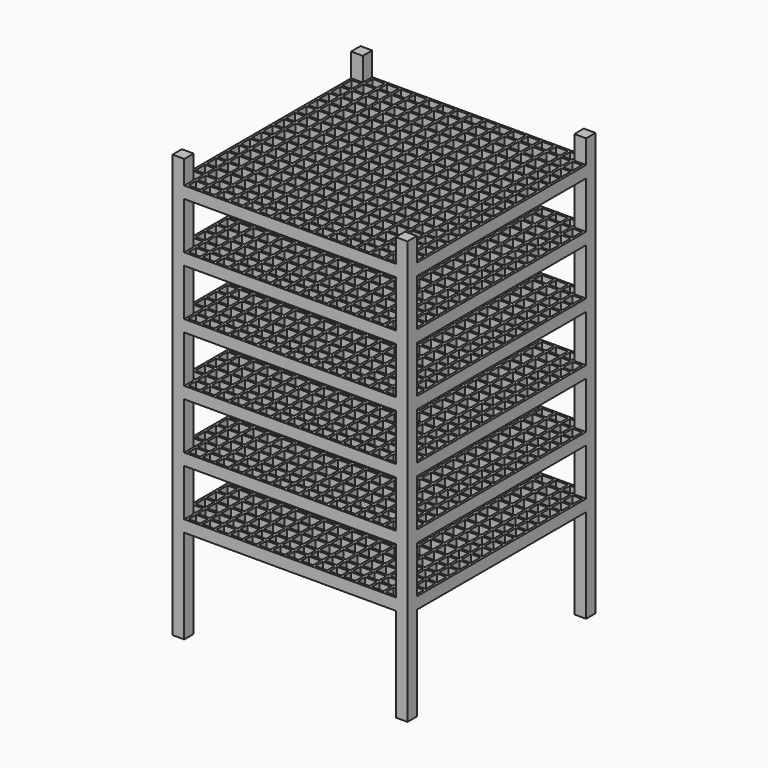
from build123d import *

# Parameters (mm, degrees)
F0_W     = 1000
F0_H     = 1000
F1_DEPTH = 1800
F2_W     = 900
F2_H     = 400
F2_H_2   = 200
F2_H_3   = 100
F4_DEPTH = 1000
F3_W     = 900
F3_H     = 400
F3_H_2   = 200
F3_H_3   = 100
F5_DEPTH = 1000
F6_W     = 40
F6_H     = 40
F6_H_2   = 50
F6_H_3   = 39.9711348116
F6_W_2   = 50
F7_DEPTH = 1800


with BuildPart() as f1:
    # F0 (on Top) → F1 (new body)
    with BuildSketch(Plane.XY):
        with Locations((-500, 500)):
            Rectangle(F0_W, F0_H)
    extrude(amount=F1_DEPTH)

    # F2 (on face) → F4 (cut)
    with BuildSketch(Plane.XZ):
        with Locations((-500, 200)):
            Rectangle(F2_W, F2_H)
        with Locations((-500, 550)):
            Rectangle(F2_W, F2_H_2)
        with Locations((-500, 800)):
            Rectangle(F2_W, F2_H_2)
        with Locations((-500, 1050)):
            Rectangle(F2_W, F2_H_2)
        with Locations((-500, 1300)):
            Rectangle(F2_W, F2_H_2)
        with Locations((-500, 1550)):
            Rectangle(F2_W, F2_H_2)
        with Locations((-500, 1750)):
            Rectangle(F2_W, F2_H_3)
    extrude(amount=-F4_DEPTH, mode=Mode.SUBTRACT)

    # F3 (on face) → F5 (cut)
    with BuildSketch(Plane.YZ):
        with Locations((500, 200)):
            Rectangle(F3_W, F3_H)
        with Locations((500, 550)):
            Rectangle(F3_W, F3_H_2)
        with Locations((500, 800)):
            Rectangle(F3_W, F3_H_2)
        with Locations((500, 1050)):
            Rectangle(F3_W, F3_H_2)
        with Locations((500, 1300)):
            Rectangle(F3_W, F3_H_2)
        with Locations((500, 1550)):
            Rectangle(F3_W, F3_H_2)
        with Locations((500, 1750)):
            Rectangle(F3_W, F3_H_3)
    extrude(amount=-F5_DEPTH, mode=Mode.SUBTRACT)

    # F6 (on face) → F7 (cut)
    with BuildSketch(Plane.XY.offset(1700)):
        with Locations((-30, 80)):
            Rectangle(F6_W, F6_H)
        with Locations((-30, 915)):
            Rectangle(F6_W, F6_H_2)
        with Locations((-30, 855)):
            Rectangle(F6_W, F6_H_2)
        with Locations((-30, 795)):
            Rectangle(F6_W, F6_H_2)
        with Locations((-30, 735)):
            Rectangle(F6_W, F6_H_2)
        with Locations((-30, 675)):
            Rectangle(F6_W, F6_H_2)
        with Locations((-30, 615)):
            Rectangle(F6_W, F6_H_2)
        with Locations((-30, 555)):
            Rectangle(F6_W, F6_H_2)
        with Locations((-30, 495)):
            Rectangle(F6_W, F6_H_2)
        with Locations((-30, 435)):
            Rectangle(F6_W, F6_H_2)
        with Locations((-30, 375)):
            Rectangle(F6_W, F6_H_2)
        with Locations((-30, 315)):
            Rectangle(F6_W, F6_H_2)
        with Locations((-30, 255)):
            Rectangle(F6_W, F6_H_2)
        with Locations((-30, 195)):
            Rectangle(F6_W, F6_H_2)
        with Locations((-30, 135)):
            Rectangle(F6_W, F6_H_2)
        with Locations((-80, 30.0144325942)):
            Rectangle(F6_W, F6_H_3)
        with Locations((-80, 80)):
            Rectangle(F6_W, F6_H)
        with Locations((-80, 135)):
            Rectangle(F6_W, F6_H_2)
        with Locations((-80, 195)):
            Rectangle(F6_W, F6_H_2)
        with Locations((-80, 255)):
            Rectangle(F6_W, F6_H_2)
        with Locations((-80, 315)):
            Rectangle(F6_W, F6_H_2)
        with Locations((-80, 375)):
            Rectangle(F6_W, F6_H_2)
        with Locations((-80, 435)):
            Rectangle(F6_W, F6_H_2)
        with Locations((-80, 495)):
            Rectangle(F6_W, F6_H_2)
        with Locations((-80, 555)):
            Rectangle(F6_W, F6_H_2)
        with Locations((-80, 615)):
            Rectangle(F6_W, F6_H_2)
        with Locations((-80, 675)):
            Rectangle(F6_W, F6_H_2)
        with Locations((-80, 735)):
            Rectangle(F6_W, F6_H_2)
        with Locations((-80, 795)):
            Rectangle(F6_W, F6_H_2)
        with Locations((-80, 855)):
            Rectangle(F6_W, F6_H_2)
        with Locations((-80, 915)):
            Rectangle(F6_W, F6_H_2)
        with Locations((-80, 970)):
            Rectangle(F6_W, F6_H)
        with Locations((-135, 970)):
            Rectangle(F6_W_2, F6_H)
        with Locations((-135, 915)):
            Rectangle(F6_W_2, F6_H_2)
        with Locations((-135, 855)):
            Rectangle(F6_W_2, F6_H_2)
        with Locations((-135, 795)):
            Rectangle(F6_W_2, F6_H_2)
        with Locations((-135, 735)):
            Rectangle(F6_W_2, F6_H_2)
        with Locations((-135, 675)):
            Rectangle(F6_W_2, F6_H_2)
        with Locations((-135, 615)):
            Rectangle(F6_W_2, F6_H_2)
        with Locations((-135, 555)):
            Rectangle(F6_W_2, F6_H_2)
        with Locations((-135, 495)):
            Rectangle(F6_W_2, F6_H_2)
        with Locations((-135, 435)):
            Rectangle(F6_W_2, F6_H_2)
        with Locations((-135, 375)):
            Rectangle(F6_W_2, F6_H_2)
        with Locations((-135, 315)):
            Rectangle(F6_W_2, F6_H_2)
        with Locations((-135, 255)):
            Rectangle(F6_W_2, F6_H_2)
        with Locations((-135, 195)):
            Rectangle(F6_W_2, F6_H_2)
        with Locations((-135, 135)):
            Rectangle(F6_W_2, F6_H_2)
        with Locations((-135, 80)):
            Rectangle(F6_W_2, F6_H)
        with Locations((-135, 30.0144325942)):
            Rectangle(F6_W_2, F6_H_3)
        with Locations((-195, 30.0144325942)):
            Rectangle(F6_W_2, F6_H_3)
        with Locations((-195, 80)):
            Rectangle(F6_W_2, F6_H)
        with Locations((-195, 135)):
            Rectangle(F6_W_2, F6_H_2)
        with Locations((-195, 195)):
            Rectangle(F6_W_2, F6_H_2)
        with Locations((-195, 255)):
            Rectangle(F6_W_2, F6_H_2)
        with Locations((-195, 315)):
            Rectangle(F6_W_2, F6_H_2)
        with Locations((-195, 375)):
            Rectangle(F6_W_2, F6_H_2)
        with Locations((-195, 435)):
            Rectangle(F6_W_2, F6_H_2)
        with Locations((-195, 495)):
            Rectangle(F6_W_2, F6_H_2)
        with Locations((-195, 555)):
            Rectangle(F6_W_2, F6_H_2)
        with Locations((-195, 615)):
            Rectangle(F6_W_2, F6_H_2)
        with Locations((-195, 675)):
            Rectangle(F6_W_2, F6_H_2)
        with Locations((-195, 735)):
            Rectangle(F6_W_2, F6_H_2)
        with Locations((-195, 795)):
            Rectangle(F6_W_2, F6_H_2)
        with Locations((-195, 855)):
            Rectangle(F6_W_2, F6_H_2)
        with Locations((-195, 915)):
            Rectangle(F6_W_2, F6_H_2)
        with Locations((-255, 970)):
            Rectangle(F6_W_2, F6_H)
        with Locations((-195, 970)):
            Rectangle(F6_W_2, F6_H)
        with Locations((-255, 915)):
            Rectangle(F6_W_2, F6_H_2)
        with Locations((-255, 855)):
            Rectangle(F6_W_2, F6_H_2)
        with Locations((-255, 795)):
            Rectangle(F6_W_2, F6_H_2)
        with Locations((-255, 735)):
            Rectangle(F6_W_2, F6_H_2)
        with Locations((-255, 675)):
            Rectangle(F6_W_2, F6_H_2)
        with Locations((-255, 615)):
            Rectangle(F6_W_2, F6_H_2)
        with Locations((-255, 555)):
            Rectangle(F6_W_2, F6_H_2)
        with Locations((-255, 495)):
            Rectangle(F6_W_2, F6_H_2)
        with Locations((-255, 435)):
            Rectangle(F6_W_2, F6_H_2)
        with Locations((-255, 375)):
            Rectangle(F6_W_2, F6_H_2)
        with Locations((-255, 315)):
            Rectangle(F6_W_2, F6_H_2)
        with Locations((-255, 255)):
            Rectangle(F6_W_2, F6_H_2)
        with Locations((-255, 195)):
            Rectangle(F6_W_2, F6_H_2)
        with Locations((-255, 135)):
            Rectangle(F6_W_2, F6_H_2)
        with Locations((-255, 80)):
            Rectangle(F6_W_2, F6_H)
        with Locations((-255, 30.0144325942)):
            Rectangle(F6_W_2, F6_H_3)
        with Locations((-315, 30.0144325942)):
            Rectangle(F6_W_2, F6_H_3)
        with Locations((-315, 80)):
            Rectangle(F6_W_2, F6_H)
        with Locations((-315, 135)):
            Rectangle(F6_W_2, F6_H_2)
        with Locations((-315, 195)):
            Rectangle(F6_W_2, F6_H_2)
        with Locations((-315, 255)):
            Rectangle(F6_W_2, F6_H_2)
        with Locations((-315, 315)):
            Rectangle(F6_W_2, F6_H_2)
        with Locations((-315, 375)):
            Rectangle(F6_W_2, F6_H_2)
        with Locations((-315, 435)):
            Rectangle(F6_W_2, F6_H_2)
        with Locations((-315, 495)):
            Rectangle(F6_W_2, F6_H_2)
        with Locations((-315, 555)):
            Rectangle(F6_W_2, F6_H_2)
        with Locations((-315, 615)):
            Rectangle(F6_W_2, F6_H_2)
        with Locations((-315, 675)):
            Rectangle(F6_W_2, F6_H_2)
        with Locations((-315, 735)):
            Rectangle(F6_W_2, F6_H_2)
        with Locations((-315, 795)):
            Rectangle(F6_W_2, F6_H_2)
        with Locations((-315, 855)):
            Rectangle(F6_W_2, F6_H_2)
        with Locations((-315, 915)):
            Rectangle(F6_W_2, F6_H_2)
        with Locations((-315, 970)):
            Rectangle(F6_W_2, F6_H)
        with Locations((-375, 970)):
            Rectangle(F6_W_2, F6_H)
        with Locations((-375, 915)):
            Rectangle(F6_W_2, F6_H_2)
        with Locations((-375, 855)):
            Rectangle(F6_W_2, F6_H_2)
        with Locations((-375, 795)):
            Rectangle(F6_W_2, F6_H_2)
        with Locations((-375, 735)):
            Rectangle(F6_W_2, F6_H_2)
        with Locations((-375, 675)):
            Rectangle(F6_W_2, F6_H_2)
        with Locations((-375, 615)):
            Rectangle(F6_W_2, F6_H_2)
        with Locations((-375, 555)):
            Rectangle(F6_W_2, F6_H_2)
        with Locations((-375, 495)):
            Rectangle(F6_W_2, F6_H_2)
        with Locations((-375, 435)):
            Rectangle(F6_W_2, F6_H_2)
        with Locations((-375, 375)):
            Rectangle(F6_W_2, F6_H_2)
        with Locations((-375, 315)):
            Rectangle(F6_W_2, F6_H_2)
        with Locations((-375, 255)):
            Rectangle(F6_W_2, F6_H_2)
        with Locations((-375, 195)):
            Rectangle(F6_W_2, F6_H_2)
        with Locations((-375, 135)):
            Rectangle(F6_W_2, F6_H_2)
        with Locations((-375, 80)):
            Rectangle(F6_W_2, F6_H)
        with Locations((-375, 30.0144325942)):
            Rectangle(F6_W_2, F6_H_3)
        with Locations((-435, 30.0144325942)):
            Rectangle(F6_W_2, F6_H_3)
        with Locations((-435, 80)):
            Rectangle(F6_W_2, F6_H)
        with Locations((-435, 135)):
            Rectangle(F6_W_2, F6_H_2)
        with Locations((-435, 195)):
            Rectangle(F6_W_2, F6_H_2)
        with Locations((-435, 255)):
            Rectangle(F6_W_2, F6_H_2)
        with Locations((-435, 315)):
            Rectangle(F6_W_2, F6_H_2)
        with Locations((-435, 375)):
            Rectangle(F6_W_2, F6_H_2)
        with Locations((-435, 435)):
            Rectangle(F6_W_2, F6_H_2)
        with Locations((-435, 495)):
            Rectangle(F6_W_2, F6_H_2)
        with Locations((-435, 555)):
            Rectangle(F6_W_2, F6_H_2)
        with Locations((-435, 615)):
            Rectangle(F6_W_2, F6_H_2)
        with Locations((-435, 675)):
            Rectangle(F6_W_2, F6_H_2)
        with Locations((-435, 735)):
            Rectangle(F6_W_2, F6_H_2)
        with Locations((-435, 795)):
            Rectangle(F6_W_2, F6_H_2)
        with Locations((-435, 855)):
            Rectangle(F6_W_2, F6_H_2)
        with Locations((-435, 915)):
            Rectangle(F6_W_2, F6_H_2)
        with Locations((-435, 970)):
            Rectangle(F6_W_2, F6_H)
        with Locations((-495, 970)):
            Rectangle(F6_W_2, F6_H)
        with Locations((-495, 915)):
            Rectangle(F6_W_2, F6_H_2)
        with Locations((-495, 855)):
            Rectangle(F6_W_2, F6_H_2)
        with Locations((-495, 795)):
            Rectangle(F6_W_2, F6_H_2)
        with Locations((-495, 735)):
            Rectangle(F6_W_2, F6_H_2)
        with Locations((-495, 675)):
            Rectangle(F6_W_2, F6_H_2)
        with Locations((-495, 615)):
            Rectangle(F6_W_2, F6_H_2)
        with Locations((-495, 555)):
            Rectangle(F6_W_2, F6_H_2)
        with Locations((-495, 495)):
            Rectangle(F6_W_2, F6_H_2)
        with Locations((-495, 435)):
            Rectangle(F6_W_2, F6_H_2)
        with Locations((-495, 375)):
            Rectangle(F6_W_2, F6_H_2)
        with Locations((-495, 315)):
            Rectangle(F6_W_2, F6_H_2)
        with Locations((-495, 255)):
            Rectangle(F6_W_2, F6_H_2)
        with Locations((-495, 195)):
            Rectangle(F6_W_2, F6_H_2)
        with Locations((-495, 80)):
            Rectangle(F6_W_2, F6_H)
        with Locations((-495, 30.0144325942)):
            Rectangle(F6_W_2, F6_H_3)
        with Locations((-555, 30.0144325942)):
            Rectangle(F6_W_2, F6_H_3)
        with Locations((-555, 80)):
            Rectangle(F6_W_2, F6_H)
        with Locations((-555, 135)):
            Rectangle(F6_W_2, F6_H_2)
        with Locations((-495, 135)):
            Rectangle(F6_W_2, F6_H_2)
        with Locations((-555, 195)):
            Rectangle(F6_W_2, F6_H_2)
        with Locations((-555, 255)):
            Rectangle(F6_W_2, F6_H_2)
        with Locations((-555, 315)):
            Rectangle(F6_W_2, F6_H_2)
        with Locations((-555, 375)):
            Rectangle(F6_W_2, F6_H_2)
        with Locations((-555, 435)):
            Rectangle(F6_W_2, F6_H_2)
        with Locations((-555, 495)):
            Rectangle(F6_W_2, F6_H_2)
        with Locations((-555, 555)):
            Rectangle(F6_W_2, F6_H_2)
        with Locations((-555, 615)):
            Rectangle(F6_W_2, F6_H_2)
        with Locations((-555, 675)):
            Rectangle(F6_W_2, F6_H_2)
        with Locations((-555, 735)):
            Rectangle(F6_W_2, F6_H_2)
        with Locations((-555, 795)):
            Rectangle(F6_W_2, F6_H_2)
        with Locations((-555, 855)):
            Rectangle(F6_W_2, F6_H_2)
        with Locations((-555, 915)):
            Rectangle(F6_W_2, F6_H_2)
        with Locations((-555, 970)):
            Rectangle(F6_W_2, F6_H)
        with Locations((-615, 970)):
            Rectangle(F6_W_2, F6_H)
        with Locations((-675, 970)):
            Rectangle(F6_W_2, F6_H)
        with Locations((-675, 915)):
            Rectangle(F6_W_2, F6_H_2)
        with Locations((-615, 915)):
            Rectangle(F6_W_2, F6_H_2)
        with Locations((-615, 855)):
            Rectangle(F6_W_2, F6_H_2)
        with Locations((-675, 855)):
            Rectangle(F6_W_2, F6_H_2)
        with Locations((-675, 795)):
            Rectangle(F6_W_2, F6_H_2)
        with Locations((-615, 795)):
            Rectangle(F6_W_2, F6_H_2)
        with Locations((-615, 735)):
            Rectangle(F6_W_2, F6_H_2)
        with Locations((-675, 735)):
            Rectangle(F6_W_2, F6_H_2)
        with Locations((-675, 675)):
            Rectangle(F6_W_2, F6_H_2)
        with Locations((-615, 675)):
            Rectangle(F6_W_2, F6_H_2)
        with Locations((-615, 615)):
            Rectangle(F6_W_2, F6_H_2)
        with Locations((-675, 615)):
            Rectangle(F6_W_2, F6_H_2)
        with Locations((-675, 555)):
            Rectangle(F6_W_2, F6_H_2)
        with Locations((-615, 555)):
            Rectangle(F6_W_2, F6_H_2)
        with Locations((-615, 495)):
            Rectangle(F6_W_2, F6_H_2)
        with Locations((-675, 495)):
            Rectangle(F6_W_2, F6_H_2)
        with Locations((-675, 435)):
            Rectangle(F6_W_2, F6_H_2)
        with Locations((-615, 435)):
            Rectangle(F6_W_2, F6_H_2)
        with Locations((-615, 375)):
            Rectangle(F6_W_2, F6_H_2)
        with Locations((-675, 375)):
            Rectangle(F6_W_2, F6_H_2)
        with Locations((-675, 315)):
            Rectangle(F6_W_2, F6_H_2)
        with Locations((-615, 315)):
            Rectangle(F6_W_2, F6_H_2)
        with Locations((-615, 255)):
            Rectangle(F6_W_2, F6_H_2)
        with Locations((-675, 255)):
            Rectangle(F6_W_2, F6_H_2)
        with Locations((-675, 195)):
            Rectangle(F6_W_2, F6_H_2)
        with Locations((-615, 195)):
            Rectangle(F6_W_2, F6_H_2)
        with Locations((-615, 135)):
            Rectangle(F6_W_2, F6_H_2)
        with Locations((-675, 135)):
            Rectangle(F6_W_2, F6_H_2)
        with Locations((-675, 80)):
            Rectangle(F6_W_2, F6_H)
        with Locations((-615, 80)):
            Rectangle(F6_W_2, F6_H)
        with Locations((-615, 30.0144325942)):
            Rectangle(F6_W_2, F6_H_3)
        with Locations((-675, 30.0144325942)):
            Rectangle(F6_W_2, F6_H_3)
        with Locations((-735, 30.0144325942)):
            Rectangle(F6_W_2, F6_H_3)
        with Locations((-735, 80)):
            Rectangle(F6_W_2, F6_H)
        with Locations((-735, 135)):
            Rectangle(F6_W_2, F6_H_2)
        with Locations((-735, 195)):
            Rectangle(F6_W_2, F6_H_2)
        with Locations((-735, 255)):
            Rectangle(F6_W_2, F6_H_2)
        with Locations((-735, 315)):
            Rectangle(F6_W_2, F6_H_2)
        with Locations((-735, 375)):
            Rectangle(F6_W_2, F6_H_2)
        with Locations((-735, 435)):
            Rectangle(F6_W_2, F6_H_2)
        with Locations((-735, 495)):
            Rectangle(F6_W_2, F6_H_2)
        with Locations((-735, 615)):
            Rectangle(F6_W_2, F6_H_2)
        with Locations((-735, 555)):
            Rectangle(F6_W_2, F6_H_2)
        with Locations((-735, 735)):
            Rectangle(F6_W_2, F6_H_2)
        with Locations((-735, 675)):
            Rectangle(F6_W_2, F6_H_2)
        with Locations((-735, 795)):
            Rectangle(F6_W_2, F6_H_2)
        with Locations((-735, 855)):
            Rectangle(F6_W_2, F6_H_2)
        with Locations((-735, 915)):
            Rectangle(F6_W_2, F6_H_2)
        with Locations((-735, 970)):
            Rectangle(F6_W_2, F6_H)
        with Locations((-795, 970)):
            Rectangle(F6_W_2, F6_H)
        with Locations((-855, 970)):
            Rectangle(F6_W_2, F6_H)
        with Locations((-915, 970)):
            Rectangle(F6_W_2, F6_H)
        with Locations((-915, 915)):
            Rectangle(F6_W_2, F6_H_2)
        with Locations((-970, 915)):
            Rectangle(F6_W, F6_H_2)
        with Locations((-970, 855)):
            Rectangle(F6_W, F6_H_2)
        with Locations((-970, 795)):
            Rectangle(F6_W, F6_H_2)
        with Locations((-915, 795)):
            Rectangle(F6_W_2, F6_H_2)
        with Locations((-915, 855)):
            Rectangle(F6_W_2, F6_H_2)
        with Locations((-855, 855)):
            Rectangle(F6_W_2, F6_H_2)
        with Locations((-855, 915)):
            Rectangle(F6_W_2, F6_H_2)
        with Locations((-795, 915)):
            Rectangle(F6_W_2, F6_H_2)
        with Locations((-795, 855)):
            Rectangle(F6_W_2, F6_H_2)
        with Locations((-795, 795)):
            Rectangle(F6_W_2, F6_H_2)
        with Locations((-855, 795)):
            Rectangle(F6_W_2, F6_H_2)
        with Locations((-855, 735)):
            Rectangle(F6_W_2, F6_H_2)
        with Locations((-795, 735)):
            Rectangle(F6_W_2, F6_H_2)
        with Locations((-795, 675)):
            Rectangle(F6_W_2, F6_H_2)
        with Locations((-855, 675)):
            Rectangle(F6_W_2, F6_H_2)
        with Locations((-855, 615)):
            Rectangle(F6_W_2, F6_H_2)
        with Locations((-795, 615)):
            Rectangle(F6_W_2, F6_H_2)
        with Locations((-795, 555)):
            Rectangle(F6_W_2, F6_H_2)
        with Locations((-855, 555)):
            Rectangle(F6_W_2, F6_H_2)
        with Locations((-855, 495)):
            Rectangle(F6_W_2, F6_H_2)
        with Locations((-795, 495)):
            Rectangle(F6_W_2, F6_H_2)
        with Locations((-795, 435)):
            Rectangle(F6_W_2, F6_H_2)
        with Locations((-855, 435)):
            Rectangle(F6_W_2, F6_H_2)
        with Locations((-855, 375)):
            Rectangle(F6_W_2, F6_H_2)
        with Locations((-795, 375)):
            Rectangle(F6_W_2, F6_H_2)
        with Locations((-795, 315)):
            Rectangle(F6_W_2, F6_H_2)
        with Locations((-855, 315)):
            Rectangle(F6_W_2, F6_H_2)
        with Locations((-855, 255)):
            Rectangle(F6_W_2, F6_H_2)
        with Locations((-795, 255)):
            Rectangle(F6_W_2, F6_H_2)
        with Locations((-795, 195)):
            Rectangle(F6_W_2, F6_H_2)
        with Locations((-855, 195)):
            Rectangle(F6_W_2, F6_H_2)
        with Locations((-855, 135)):
            Rectangle(F6_W_2, F6_H_2)
        with Locations((-795, 135)):
            Rectangle(F6_W_2, F6_H_2)
        with Locations((-795, 80)):
            Rectangle(F6_W_2, F6_H)
        with Locations((-855, 80)):
            Rectangle(F6_W_2, F6_H)
        with Locations((-855, 30.0144325942)):
            Rectangle(F6_W_2, F6_H_3)
        with Locations((-795, 30.0144325942)):
            Rectangle(F6_W_2, F6_H_3)
        with Locations((-915, 30.0144325942)):
            Rectangle(F6_W_2, F6_H_3)
        with Locations((-915, 80)):
            Rectangle(F6_W_2, F6_H)
        with Locations((-970, 80)):
            Rectangle(F6_W, F6_H)
        with Locations((-970, 135)):
            Rectangle(F6_W, F6_H_2)
        with Locations((-915, 135)):
            Rectangle(F6_W_2, F6_H_2)
        with Locations((-915, 195)):
            Rectangle(F6_W_2, F6_H_2)
        with Locations((-970, 195)):
            Rectangle(F6_W, F6_H_2)
        with Locations((-970, 255)):
            Rectangle(F6_W, F6_H_2)
        with Locations((-915, 255)):
            Rectangle(F6_W_2, F6_H_2)
        with Locations((-915, 315)):
            Rectangle(F6_W_2, F6_H_2)
        with Locations((-970, 315)):
            Rectangle(F6_W, F6_H_2)
        with Locations((-970, 375)):
            Rectangle(F6_W, F6_H_2)
        with Locations((-915, 375)):
            Rectangle(F6_W_2, F6_H_2)
        with Locations((-915, 435)):
            Rectangle(F6_W_2, F6_H_2)
        with Locations((-970, 435)):
            Rectangle(F6_W, F6_H_2)
        with Locations((-970, 495)):
            Rectangle(F6_W, F6_H_2)
        with Locations((-915, 495)):
            Rectangle(F6_W_2, F6_H_2)
        with Locations((-915, 555)):
            Rectangle(F6_W_2, F6_H_2)
        with Locations((-970, 555)):
            Rectangle(F6_W, F6_H_2)
        with Locations((-970, 615)):
            Rectangle(F6_W, F6_H_2)
        with Locations((-915, 615)):
            Rectangle(F6_W_2, F6_H_2)
        with Locations((-915, 675)):
            Rectangle(F6_W_2, F6_H_2)
        with Locations((-970, 675)):
            Rectangle(F6_W, F6_H_2)
        with Locations((-970, 735)):
            Rectangle(F6_W, F6_H_2)
        with Locations((-915, 735)):
            Rectangle(F6_W_2, F6_H_2)
    extrude(amount=-F7_DEPTH, mode=Mode.SUBTRACT)


solid = f1.part
